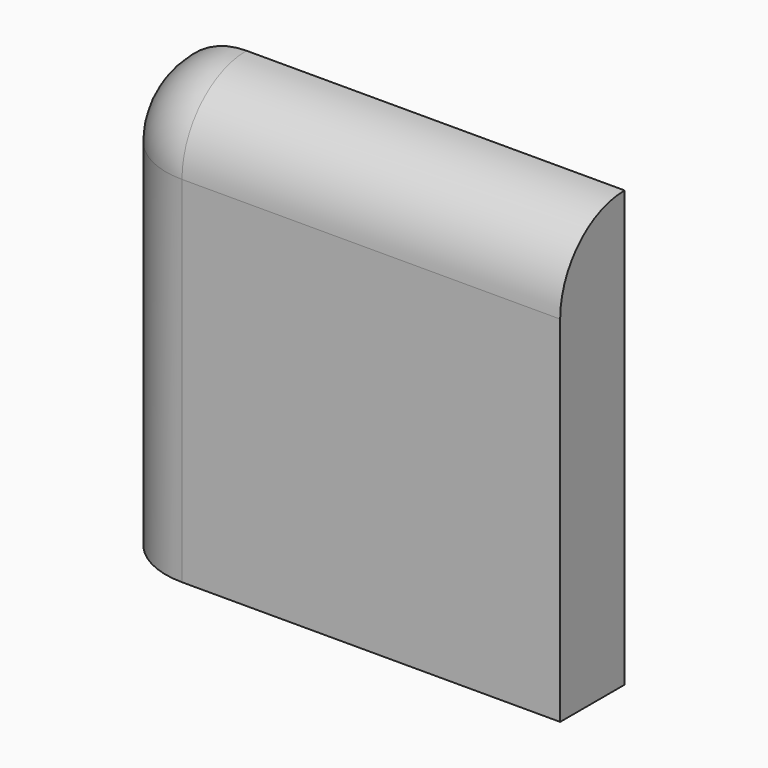
from build123d import *

# Parameters (mm, degrees)
F0_W     = 144.6518152952
F0_H     = 137.2342258692
F2_DEPTH = 25.4
F1_R     = 25.39999


# Not quite as in the source:
# - a fillet or chamfer is up to 0.001 mm smaller than in the source, because OpenCascade refuses the exact size


with BuildPart() as f2:
    # F0 (on Front) → F2 (new body)
    with BuildSketch(Plane.XZ):
        with Locations((23.3432799578, -12.742228806)):
            Rectangle(F0_W, F0_H)
    extrude(amount=F2_DEPTH)

    # F1 (radius 25.4 in the source; OpenCascade refuses exactly that, so slightly less here)
    f1_edges = [f2.edges().sort_by_distance(p)[0] for p in [
        (-48.982628, -12.7, 55.874884),
        (23.34328, -25.4, 55.874884),
        (-48.982628, -25.4, -12.742229),
    ]]
    fillet(f1_edges, radius=F1_R)


solid = f2.part
